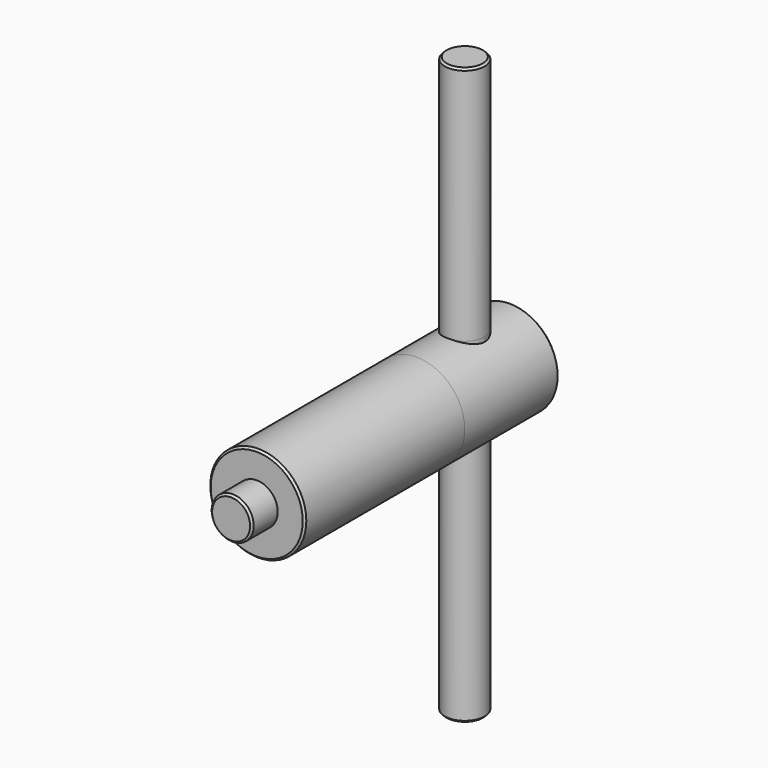
from build123d import *

# Parameters (mm, degrees)
F0_R          = 12
F1_DEPTH      = 20
F2_R          = 12
F3_DEPTH      = 10
F6_R          = 5
F7_DEPTH      = 60
F7_DEPTH_BACK = 3
F8_R          = 5
F9_DEPTH      = 60
F9_DEPTH_BACK = 3
F10_SIZE      = 1
F11_SIZE      = 0.5
F12_R         = 12
F13_DEPTH     = 50
F14_R         = 5.25
F15_DEPTH     = 8
F16_SIZE      = 0.5


with BuildPart() as f1:
    # F0 (on Front) → F1 (new body)
    with BuildSketch(Plane.XZ):
        Circle(F0_R)
    extrude(amount=F1_DEPTH)

    # F2 (on face) → F3 (join)
    with BuildSketch(Plane.XZ.offset(20)):
        Circle(F2_R)
    extrude(amount=F3_DEPTH)

    # F6 (on offset) → F7 (join, two sides)
    with BuildSketch(Plane.XY.offset(12)) as f7_sk:
        with Locations((0, -15)):
            Circle(F6_R)
    extrude(amount=F7_DEPTH)
    extrude(f7_sk.sketch, amount=-F7_DEPTH_BACK)

    # F8 (on offset) → F9 (join, two sides)
    with BuildSketch(Plane.XY.offset(-12)) as f9_sk:
        with Locations((0, -15)):
            Circle(F8_R)
    extrude(amount=-F9_DEPTH)
    extrude(f9_sk.sketch, amount=F9_DEPTH_BACK)

    # F10
    f10_edges = [f1.edges().sort_by_distance(p)[0] for p in [
        (-12, 0, 0),
    ]]
    chamfer(f10_edges, length=F10_SIZE)

    # F11
    f11_edges = [f1.edges().sort_by_distance(p)[0] for p in [
        (-5, -15, 72),
        (-5, -15, -72),
    ]]
    chamfer(f11_edges, length=F11_SIZE)


with BuildPart() as f13:
    # F12 (on face) → F13 (new body)
    with BuildSketch(Plane.XZ.offset(30)):
        Circle(F12_R)
    extrude(amount=F13_DEPTH)

    # F14 (on face) → F15 (join)
    with BuildSketch(Plane.XZ.offset(80)):
        Circle(F14_R)
    extrude(amount=F15_DEPTH)

    # F16
    f16_edges = [f13.edges().sort_by_distance(p)[0] for p in [
        (-12, -80, 0),
        (-5.25, -88, 0),
    ]]
    chamfer(f16_edges, length=F16_SIZE)


solid = Compound([f1.part, f13.part])
